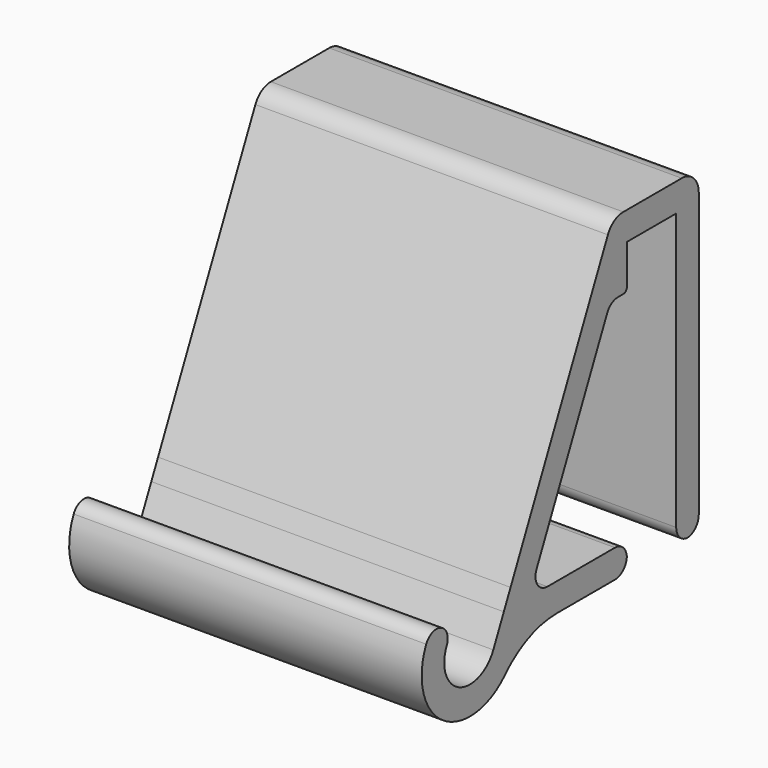
from build123d import *

# Parameters (mm, degrees)
F1_DEPTH    = 40
F2_R        = 2.4142135624
F3_R        = 10.2321597652
F4_T1_DEPTH = 40
F4_T3_DEPTH = 48.4497474683
F5_R        = 0.5


# Not quite as in the source:
# - a fillet or chamfer that OpenCascade refuses, or shapes differently, is made with other operations: its cross-section is extruded or revolved along the edge and cut away or added


with BuildPart() as f1:
    # F0 (on Right) → F1 (new body)
    with BuildSketch(Plane.YZ):
        with BuildLine():
            ThreePointArc((-25.4094946088, 3.7613025295), (-26.6631912182, 5.323376139), (-28.4595870608, 4.4374917638))
            ThreePointArc((-28.4595870608, 4.4374917638), (-27.6856838354, 2.3112100739), (-25.5594021496, 3.0851133107))
            ThreePointArc((-25.5594021496, 3.0851133107), (-25.4474209974, 3.4149991472), (-25.4094946088, 3.7613025295))
        make_face()
        with BuildLine():
            ThreePointArc((-16.0431703857, -1.3523784376), (-15.774850852, -0.6883818658), (-15.577323066, 0))
            Line((-15.577323066, 0), (-18.9433553042, 0))
            ThreePointArc((-18.9433553042, 0), (-23.7939353822, -1.7654667673), (-25.5594021496, 3.0851133107))
            ThreePointArc((-25.5594021496, 3.0851133107), (-27.6856838354, 2.3112100739), (-28.4595870608, 4.4374917638))
            ThreePointArc((-28.4595870608, 4.4374917638), (-25.1463138276, -4.6656516822), (-16.0431703857, -1.3523784376))
        make_face()
        with BuildLine():
            ThreePointArc((-15.4013787269, 1.5425566554), (-15.4524550708, 2.3775040298), (-15.604922411, 3.2))
            Line((-15.604922411, 3.2), (-17.4511707981, 3.2))
            Line((-17.4511707981, 3.2), (-18.9433553042, 0))
            Line((-18.9433553042, 0), (-15.577323066, 0))
            ThreePointArc((-15.577323066, 0), (-15.4455069504, 0.7662774779), (-15.4013787269, 1.5425566554))
        make_face()
        with BuildLine():
            Line((-15.4125459635, 0), (-13.9203614574, 3.2))
            Line((-13.9203614574, 3.2), (-15.604922411, 3.2))
            ThreePointArc((-15.604922411, 3.2), (-15.4524550708, 2.3775040298), (-15.4013787269, 1.5425566554))
            ThreePointArc((-15.4013787269, 1.5425566554), (-15.4455069504, 0.7662774779), (-15.577323066, 0))
            Line((-15.577323066, 0), (-15.4125459635, 0))
        make_face()
        Polygon((-2.0386248346, 0), (0, 0), (0, 3.2), (-13.9203614574, 3.2), (-15.4125459635, 0), align=None)
        with BuildLine():
            Line((-15.604922411, 3.2), (-13.9203614574, 3.2))
            Line((-13.9203614574, 3.2), (-2.3315382908, 28.0523114815))
            Line((-2.3315382908, 28.0523114815), (0, 33.0523114815))
            Line((0, 33.0523114815), (7, 33.0523114815))
            Line((7, 33.0523114815), (7, 0))
            Line((7, 0), (10.2, 0))
            Line((10.2, 0), (10.2, 36.2523114815))
            Line((10.2, 36.2523114815), (-2.0386248346, 36.2523114815))
            Line((-2.0386248346, 36.2523114815), (-16.4936271239, 5.253459036))
            ThreePointArc((-16.4936271239, 5.253459036), (-15.9648640306, 4.2632611548), (-15.604922411, 3.2))
        make_face()
        with BuildLine():
            Line((-16.0431703857, -1.3523784376), (-15.4125459635, 0))
            Line((-15.4125459635, 0), (-15.577323066, 0))
            ThreePointArc((-15.577323066, 0), (-15.774850852, -0.6883818658), (-16.0431703857, -1.3523784376))
        make_face()
        with BuildLine():
            Line((-17.4511707981, 3.2), (-15.604922411, 3.2))
            ThreePointArc((-15.604922411, 3.2), (-15.9648640306, 4.2632611548), (-16.4936271239, 5.253459036))
            Line((-16.4936271239, 5.253459036), (-17.4511707981, 3.2))
        make_face()
        Polygon((-2.3315382908, 28.0523114815), (0, 28.0523114815), (0, 33.0523114815), align=None)
    extrude(amount=F1_DEPTH)

    # F2
    f2_edges = [f1.edges().sort_by_distance(p)[0] for p in [
        (20, -2.038625, 36.252311),
        (20, 10.2, 36.252311),
    ]]
    fillet(f2_edges, radius=F2_R)

    # F3
    f3_edges = [f1.edges().sort_by_distance(p)[0] for p in [
        (20, -15.412546, 0),
    ]]
    fillet(f3_edges, radius=F3_R)

    # F4: fillet of radius 1.6899494937 on 6 edges, made by hand

    # F4_s2 → F4_t1 (join)
    with BuildSketch(Plane.YZ):
        with BuildLine():
            ThreePointArc((-11.2676721112, 3.2), (-12.692961058, 3.9819402926), (-12.799286497, 5.6041530111))
            Line((-12.799286497, 5.6041530111), (-13.9203614574, 3.2))
            Line((-13.9203614574, 3.2), (-11.2676721112, 3.2))
        make_face()
        with BuildLine():
            ThreePointArc((-2.7865361119, 27.0765655052), (-2.1629309272, 27.7876509346), (-1.2549217261, 28.0523114815))
            Line((-1.2549217261, 28.0523114815), (-2.3315382908, 28.0523114815))
            Line((-2.3315382908, 28.0523114815), (-2.7865361119, 27.0765655052))
        make_face()
    extrude(amount=F4_T1_DEPTH)

    # F4_s4 → F4_t3 (cut)
    with BuildSketch(Plane.YZ.offset(-4.2248737342)):
        with BuildLine():
            ThreePointArc((8.6899494937, 0), (7.4949747468, 0.4949747468), (7, 1.6899494937))
            Line((7, 1.6899494937), (7, 0))
            Line((7, 0), (8.6899494937, 0))
        make_face()
        with BuildLine():
            ThreePointArc((0, 1.5100505063), (-0.4949747468, 2.7050252532), (-1.6899494937, 3.2))
            Line((-1.6899494937, 3.2), (0, 3.2))
            Line((0, 3.2), (0, 1.5100505063))
        make_face()
        with BuildLine():
            ThreePointArc((-1.6899494937, 0), (-0.4949747468, 0.4949747468), (0, 1.6899494937))
            Line((0, 1.6899494937), (0, 0))
            Line((0, 0), (-1.6899494937, 0))
        make_face()
        with BuildLine():
            ThreePointArc((10.2, 1.6899494937), (9.7050252532, 0.4949747468), (8.5100505063, 0))
            Line((8.5100505063, 0), (10.2, 0))
            Line((10.2, 0), (10.2, 1.6899494937))
        make_face()
    extrude(amount=F4_T3_DEPTH, mode=Mode.SUBTRACT)

    # F5
    f5_edges = [f1.edges().sort_by_distance(p)[0] for p in [
        (20, 0, 28.052311),
    ]]
    fillet(f5_edges, radius=F5_R)


solid = f1.part
